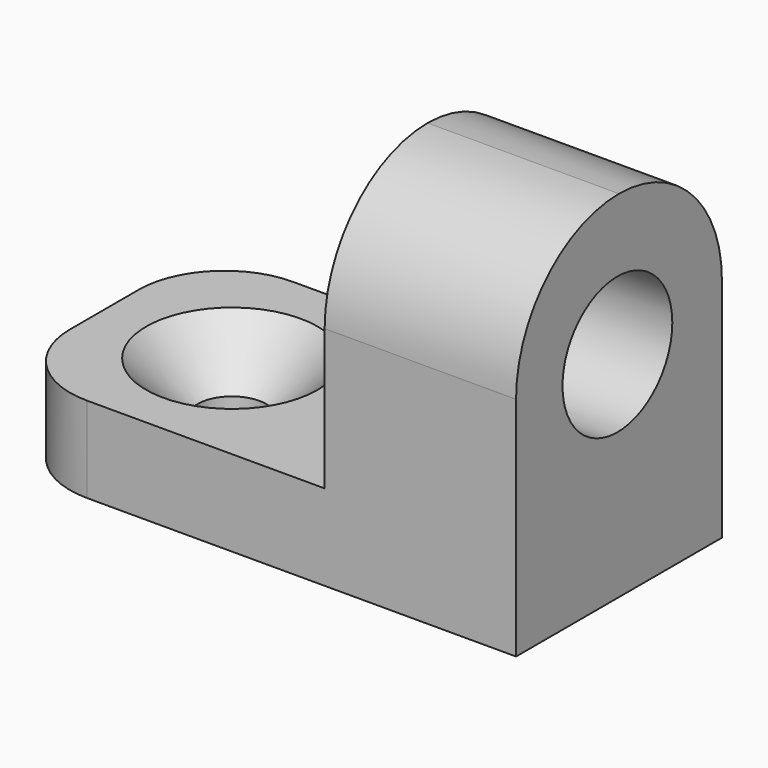
from build123d import *

# Parameters (mm, degrees)
F0_W     = 18.8419777411
F0_H     = 15
F0_R     = 2
F0_W_2   = 11.1580222589
F1_DEPTH = 5
F2_SIZE  = 3
F3_DEPTH = 20.7
F4_R     = 4
F5_DEPTH = 55.3
F6_R     = 7.49999
F7_R     = 5


# Not quite as in the source:
# - a fillet or chamfer is up to 0.001 mm smaller than in the source, because OpenCascade refuses the exact size


with BuildPart() as f1:
    # F0 (on Top) → F1 (new body)
    with BuildSketch(Plane.XY):
        with Locations((9.4734227529, 0.1149109378)):
            Rectangle(F0_W, F0_H)
        with Locations((7.5819236226, 0)):
            Circle(F0_R, mode=Mode.SUBTRACT)
        with Locations((24.4734227529, 0.1149109378)):
            Rectangle(F0_W_2, F0_H)
    extrude(amount=F1_DEPTH)

    # F2
    f2_edges = [f1.edges().sort_by_distance(p)[0] for p in [
        (5.581924, 0, 5),
    ]]
    chamfer(f2_edges, length=F2_SIZE)

    # F0 (on Top) → F3 (join)
    with BuildSketch(Plane.XY):
        with Locations((24.4734227529, 0.1149109378)):
            Rectangle(F0_W_2, F0_H)
    extrude(amount=F3_DEPTH)

    # F4 (on Right) → F5 (cut)
    with BuildSketch(Plane.YZ):
        with Locations((0, 12.5060472637)):
            Circle(F4_R)
    extrude(amount=F5_DEPTH, mode=Mode.SUBTRACT)

    # F6 (radius 7.5 in the source; OpenCascade refuses exactly that, so slightly less here)
    f6_edges = [f1.edges().sort_by_distance(p)[0] for p in [
        (24.473423, -7.385089, 20.7),
        (24.473423, 7.614911, 20.7),
    ]]
    fillet(f6_edges, radius=F6_R)

    # F7
    f7_edges = [f1.edges().sort_by_distance(p)[0] for p in [
        (0.052434, -7.385089, 2.5),
        (0.052434, 7.614911, 2.5),
    ]]
    fillet(f7_edges, radius=F7_R)


solid = f1.part
